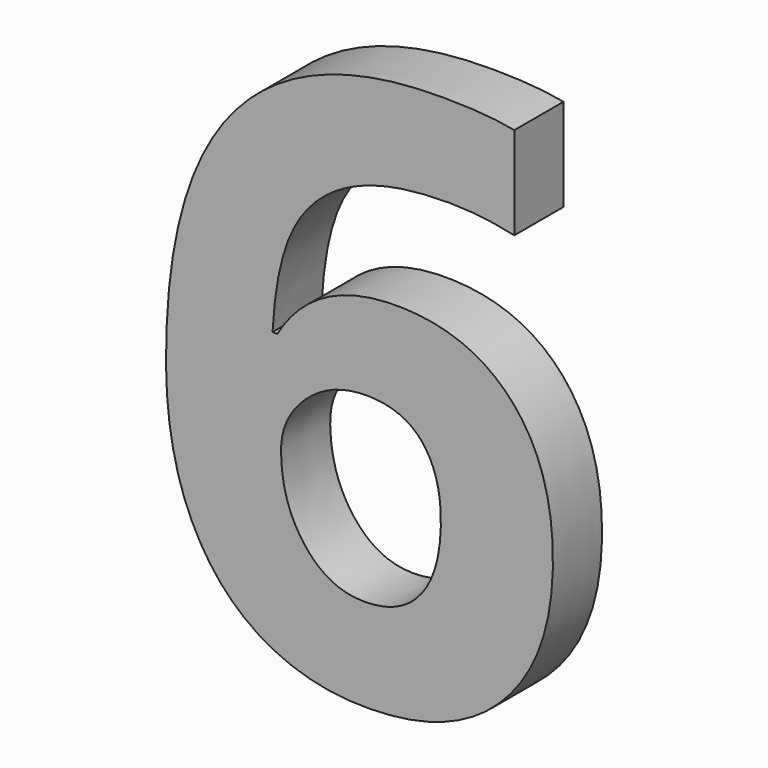
from build123d import *

# Parameters (mm, degrees)
F0_TEXT_SIZE = 62.5
F1_DEPTH     = 5


# Not quite as in the source:
# - Text() gives the source's letters only with a copy of the font that has no kerning and outlines rounded to 1/6400 em; it was checked with that copy


with BuildPart() as f1:
    # F0 (on Front) → F1 (new body)
    with BuildSketch(Plane.XZ):
        with Locations((-64.9615392145, 21.5769217051)):
            Text('6', F0_TEXT_SIZE, font='Open Sans', font_style=FontStyle.BOLD, text_align=(TextAlign.LEFT, TextAlign.BOTTOM))
    extrude(amount=F1_DEPTH)


solid = f1.part
